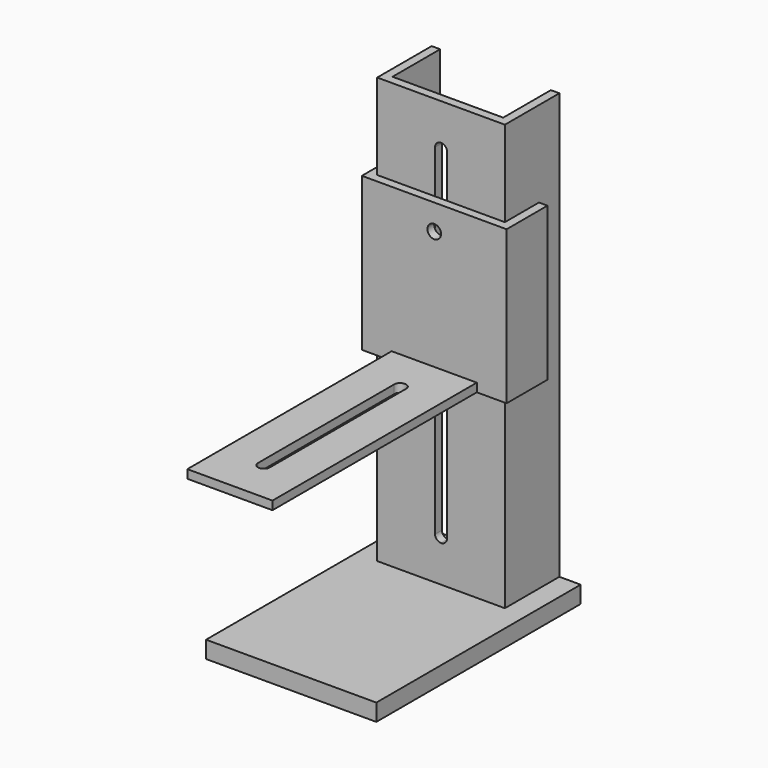
from build123d import *

# Parameters (mm, degrees)
F0_W      = 100
F0_H      = 10
F1_DEPTH  = 75
F3_DEPTH  = 250
F5_DEPTH  = 25
F6_W      = 5
F6_H      = 90
F6_W_2    = 75
F6_R      = 4
F7_DEPTH  = 5
F8_W      = 5
F8_H      = 90
F9_DEPTH  = 25
F11_DEPTH = 150
F13_DEPTH = 25


with BuildPart() as f1:
    # F0 (on Front) → F1 (new body, symmetric)
    with BuildSketch(Plane.XZ):
        Rectangle(F0_W, F0_H)
    extrude(amount=F1_DEPTH, both=True)

    # F2 (on face) → F3 (join)
    with BuildSketch(Plane.XY.offset(5)):
        Polygon((-32.5, 75), (-37.5, 75), (-37.5, 35), (0, 35), (37.5, 35), (37.5, 75), (32.5, 75), (32.5, 40), (-32.5, 40), align=None)
    extrude(amount=F3_DEPTH)

    # F4 (on face) → F5 (cut)
    with BuildSketch(Plane.XZ.offset(-35)):
        with BuildLine():
            ThreePointArc((-3.5, 30), (-2.4748737342, 27.5251262658), (0, 26.5))
            ThreePointArc((0, 26.5), (2.4748737342, 27.5251262658), (3.5, 30))
            Line((3.5, 30), (3.5, 230))
            ThreePointArc((3.5, 230), (0, 233.5), (-3.5, 230))
            Line((-3.5, 230), (-3.5, 30))
        make_face()
    extrude(amount=-F5_DEPTH, mode=Mode.SUBTRACT)


with BuildPart() as f7:
    # F6 (on face) → F7 (new body)
    with BuildSketch(Plane.XZ.offset(-35)):
        with Locations((40, 159.6051809192)):
            Rectangle(F6_W, F6_H)
        with Locations((0, 159.6051809192)):
            Rectangle(F6_W_2, F6_H)
        with Locations((0, 189.6051809192)):
            Circle(F6_R, mode=Mode.SUBTRACT)
        with Locations((-40, 159.6051809192)):
            Rectangle(F6_W, F6_H)
    extrude(amount=F7_DEPTH)

    # F8 (on face) → F9 (join)
    with BuildSketch(Plane(origin=(0, 35, 0), x_dir=(-1, 0, 0), z_dir=(0, 1, 0))):
        with Locations((-40, 159.6051809192)):
            Rectangle(F8_W, F8_H)
        with Locations((40, 159.6051809192)):
            Rectangle(F8_W, F8_H)
    extrude(amount=F9_DEPTH)

    # F10 (on face) → F11 (join)
    with BuildSketch(Plane.XZ.offset(-30)):
        Polygon((25, 119.6051809192), (0, 119.6051809192), (-25, 119.6051809192), (-25, 114.6051809192), (25, 114.6051809192), align=None)
    extrude(amount=F11_DEPTH)

    # F12 (on face) → F13 (cut)
    with BuildSketch(Plane.XY.offset(119.6051809192)):
        with BuildLine():
            ThreePointArc((-3.5, -95), (0, -98.5), (3.5, -95))
            Line((3.5, -95), (3.5, 5))
            ThreePointArc((3.5, 5), (0, 8.5), (-3.5, 5))
            Line((-3.5, 5), (-3.5, -95))
        make_face()
    extrude(amount=-F13_DEPTH, mode=Mode.SUBTRACT)


solid = Compound([f1.part, f7.part])
